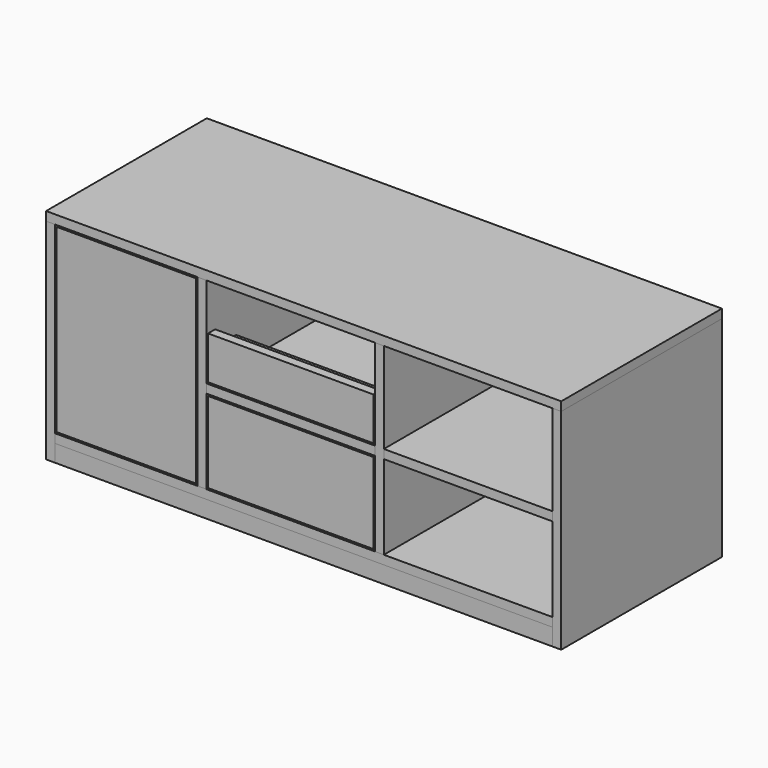
from build123d import *

# Parameters (mm, degrees)
F3_DEPTH  = 393.7
F4_DEPTH  = 393.7
F5_DEPTH  = 393.7
F6_DEPTH  = 393.7
F7_DEPTH  = 393.7
F8_START  = -17.4625
F2_W      = 279.4
F2_H      = 17.4625
F8_DEPTH  = 376.2375
F9_DEPTH  = 393.7
F2_W_2    = 974.725
F2_H_2    = 33.3375
F10_DEPTH = 17.4625
F2_W_3    = 330.2
F11_DEPTH = 393.7
F12_DEPTH = 393.7
F13_W     = 323.85
F13_H     = 158.75
F14_DEPTH = 17.4625
F15_W     = 17.4625
F15_H     = 152.4
F16_DEPTH = 358.775
F17_W     = 304.8
F17_H     = 152.4
F18_DEPTH = 17.4625
F19_W     = 273.05
F19_H     = 354.0125
F20_DEPTH = 17.4625
F21_W     = 323.85
F21_H     = 84.1375
F22_DEPTH = 17.4625
F23_W     = 269.875
F23_H     = 152.4
F24_DEPTH = 17.4625
F25_W     = 17.4625
F25_H     = 76.2
F26_DEPTH = 358.775
F27_W     = 269.875
F27_H     = 76.2
F28_DEPTH = 17.4625
F29_W     = 304.8
F29_H     = 76.2
F30_DEPTH = 17.4625


# Not quite as in the source:
# - a variable given as a bare number and used for a length is read in inches; the dataset says mm whatever the document's units were


with BuildPart() as f3:
    # F2 (on Front) → F3 (new body)
    with BuildSketch(Plane.XZ):
        Polygon((0, 428.625), (0, 411.1625), (17.4625, 411.1625), (296.8625, 411.1625), (314.325, 411.1625), (644.525, 411.1625), (661.9875, 411.1625), (992.1875, 411.1625), (1009.65, 411.1625), (1009.65, 428.625), align=None)
    extrude(amount=-F3_DEPTH)


with BuildPart() as f4:
    # F2 (on Front) → F4 (new body)
    with BuildSketch(Plane.XZ):
        Polygon((0, 411.1625), (0, 0), (17.4625, 0), (17.4625, 33.3375), (17.4625, 50.8), (17.4625, 279.4), (17.4625, 296.8625), (17.4625, 411.1625), align=None)
    extrude(amount=-F4_DEPTH)


with BuildPart() as f5:
    # F2 (on Front) → F5 (new body)
    with BuildSketch(Plane.XZ):
        Polygon((314.325, 411.1625), (296.8625, 411.1625), (296.8625, 296.8625), (296.8625, 279.4), (296.8625, 50.8), (314.325, 50.8), (314.325, 215.9), (314.325, 233.3625), (314.325, 322.2625), align=None)
    extrude(amount=-F5_DEPTH)


with BuildPart() as f6:
    # F2 (on Front) → F6 (new body)
    with BuildSketch(Plane.XZ):
        Polygon((644.525, 50.8), (661.9875, 50.8), (661.9875, 215.9), (661.9875, 233.3625), (661.9875, 322.2625), (661.9875, 411.1625), (644.525, 411.1625), (644.525, 322.2625), (644.525, 233.3625), (644.525, 215.9), align=None)
    extrude(amount=-F6_DEPTH)


with BuildPart() as f7:
    # F2 (on Front) → F7 (new body)
    with BuildSketch(Plane.XZ):
        Polygon((992.1875, 33.3375), (992.1875, 0), (1009.65, 0), (1009.65, 411.1625), (992.1875, 411.1625), (992.1875, 322.2625), (992.1875, 233.3625), (992.1875, 215.9), (992.1875, 50.8), align=None)
    extrude(amount=-F7_DEPTH)


with BuildPart() as f8:
    # F2 (on Front) → F8 (new body)
    with BuildSketch(Plane.XZ.offset(F8_START)):
        with Locations((157.1625, 288.13125)):
            Rectangle(F2_W, F2_H)
    extrude(amount=-F8_DEPTH)


with BuildPart() as f9:
    # F2 (on Front) → F9 (new body)
    with BuildSketch(Plane.XZ):
        Polygon((17.4625, 50.8), (17.4625, 33.3375), (992.1875, 33.3375), (992.1875, 50.8), (661.9875, 50.8), (644.525, 50.8), (314.325, 50.8), (296.8625, 50.8), align=None)
    extrude(amount=-F9_DEPTH)


with BuildPart() as f10:
    # F2 (on Front) → F10 (new body)
    with BuildSketch(Plane.XZ):
        with Locations((504.825, 16.66875)):
            Rectangle(F2_W_2, F2_H_2)
    extrude(amount=-F10_DEPTH)


with BuildPart() as f11:
    # F2 (on Front) → F11 (new body)
    with BuildSketch(Plane.XZ):
        with Locations((479.425, 224.63125)):
            Rectangle(F2_W_3, F2_H)
    extrude(amount=-F11_DEPTH)


with BuildPart() as f12:
    # F2 (on Front) → F12 (new body)
    with BuildSketch(Plane.XZ):
        with Locations((827.0875, 224.63125)):
            Rectangle(F2_W_3, F2_H)
    extrude(amount=-F12_DEPTH)


with BuildPart() as f14:
    # F13 (on Front) → F14 (new body)
    with BuildSketch(Plane.XZ):
        with Locations((479.425, 133.35)):
            Rectangle(F13_W, F13_H)
    extrude(amount=-F14_DEPTH)


with BuildPart() as f16:
    # F15 (on face) → F16 (new body)
    with BuildSketch(Plane(origin=(0, 17.4625, 0), x_dir=(-1, 0, 0), z_dir=(0, 1, 0))):
        with Locations((-623.09375, 130.175)):
            Rectangle(F15_W, F15_H)
    extrude(amount=F16_DEPTH)


with BuildPart() as f18:
    # F17 (on face) → F18 (new body)
    with BuildSketch(Plane(origin=(0, 376.2375, 0), x_dir=(-1, 0, 0), z_dir=(0, 1, 0))):
        with Locations((-479.425, 130.175)):
            Rectangle(F17_W, F17_H)
    extrude(amount=F18_DEPTH)


with BuildPart() as f20:
    # F19 (on Front) → F20 (new body)
    with BuildSketch(Plane.XZ):
        with Locations((157.1625, 230.98125)):
            Rectangle(F19_W, F19_H)
    extrude(amount=-F20_DEPTH)


with BuildPart() as f22:
    # F21 (on Front) → F22 (new body)
    with BuildSketch(Plane.XZ):
        with Locations((479.425, 278.60625)):
            Rectangle(F21_W, F21_H)
    extrude(amount=-F22_DEPTH)


with BuildPart() as f24:
    # F23 (on face) → F24 (new body)
    with BuildSketch(Plane(origin=(0, 17.4625, 0), x_dir=(-1, 0, 0), z_dir=(0, 1, 0))):
        with Locations((-479.425, 130.175)):
            Rectangle(F23_W, F23_H)
    extrude(amount=F24_DEPTH)


with BuildPart() as f26:
    # F25 (on face) → F26 (new body)
    with BuildSketch(Plane(origin=(0, 17.4625, 0), x_dir=(-1, 0, 0), z_dir=(0, 1, 0))):
        with Locations((-623.09375, 274.6375)):
            Rectangle(F25_W, F25_H)
    extrude(amount=F26_DEPTH)


with BuildPart() as f28:
    # F27 (on face) → F28 (new body)
    with BuildSketch(Plane(origin=(0, 17.4625, 0), x_dir=(-1, 0, 0), z_dir=(0, 1, 0))):
        with Locations((-479.425, 274.6375)):
            Rectangle(F27_W, F27_H)
    extrude(amount=F28_DEPTH)


with BuildPart() as f30:
    # F29 (on face) → F30 (new body)
    with BuildSketch(Plane(origin=(0, 376.2375, 0), x_dir=(-1, 0, 0), z_dir=(0, 1, 0))):
        with Locations((-479.425, 274.6375)):
            Rectangle(F29_W, F29_H)
    extrude(amount=F30_DEPTH)


solid = Compound([f3.part, f4.part, f5.part, f6.part, f7.part, f8.part, f9.part, f10.part, f11.part, f12.part, f14.part, f16.part, f18.part, f20.part, f22.part, f24.part, f26.part, f28.part, f30.part])
